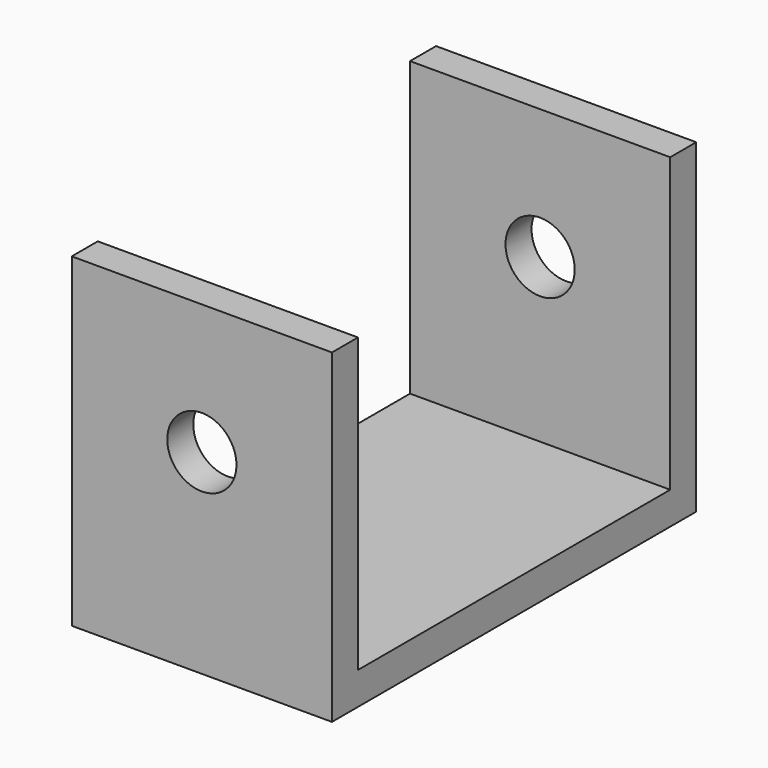
from build123d import *

# Parameters (mm, degrees)
F1_DEPTH = 12.7
F3_D     = 6.7564


with BuildPart() as f1:
    # F0 (on Right) → F1 (new body, symmetric)
    with BuildSketch(Plane.YZ):
        Polygon((-22.225, 31.75), (-22.225, 0), (0, 0), (0, 3.175), (-19.05, 3.175), (-19.05, 31.75), align=None)
        Polygon((0, 3.175), (0, 0), (22.225, 0), (22.225, 31.75), (19.05, 31.75), (19.05, 3.175), align=None)
    extrude(amount=F1_DEPTH, both=True)

    # F3 (through all)
    with Locations(Plane.XZ.offset(22.225)):
        with Locations((0, 19.05)):
            Hole(F3_D / 2)


solid = f1.part
